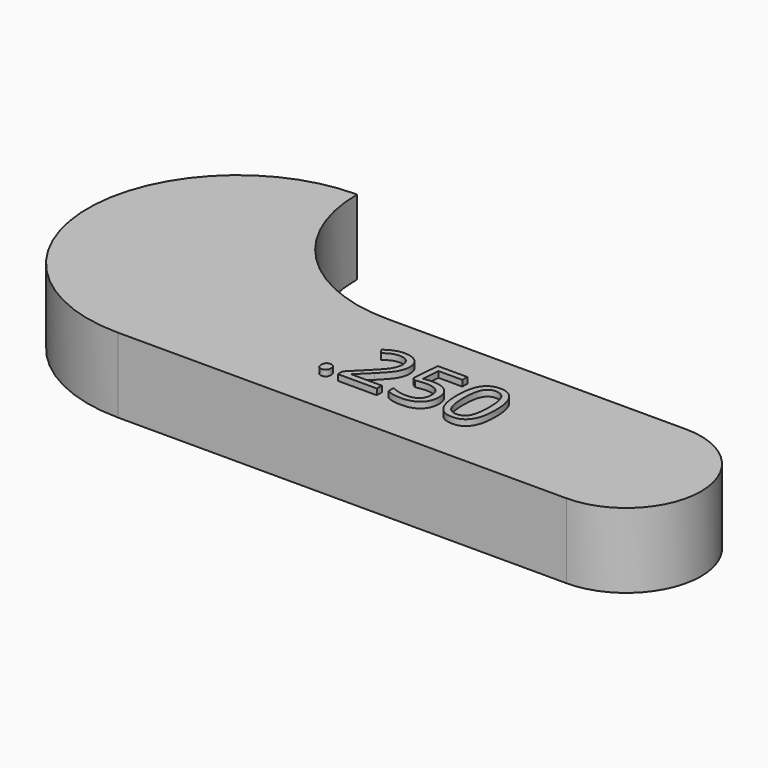
from build123d import *

# Parameters (mm, degrees)
F1_DEPTH     = 3.175
F2_TEXT_SIZE = 3.5277777778
F3_DEPTH     = 0.254


# Not quite as in the source:
# - Text() gives the source's letters only with a copy of the font that has no kerning and outlines rounded to 1/6400 em; it was checked with that copy


with BuildPart() as f1:
    # F0 (on Top) → F1 (new body)
    with BuildSketch(Plane.XY):
        with BuildLine():
            ThreePointArc((-12.7, 3.175), (-17.1901280605, 5.0348719395), (-19.05, 9.525))
            ThreePointArc((-19.05, 9.525), (-25.4, 3.175), (-19.05, -3.175))
            Line((-19.05, -3.175), (0, -3.175))
            ThreePointArc((0, -3.175), (3.175, 0), (0, 3.175))
            Line((0, 3.175), (-12.7, 3.175))
        make_face()
    extrude(amount=F1_DEPTH)

    # F2 (on face) → F3 (join)
    with BuildSketch(Plane.XY.offset(3.175)):
        with Locations((-12.2998341874, -1.3249416176)):
            Text('.250', F2_TEXT_SIZE, font='Open Sans', text_align=(TextAlign.LEFT, TextAlign.BOTTOM))
    extrude(amount=F3_DEPTH)


solid = f1.part
